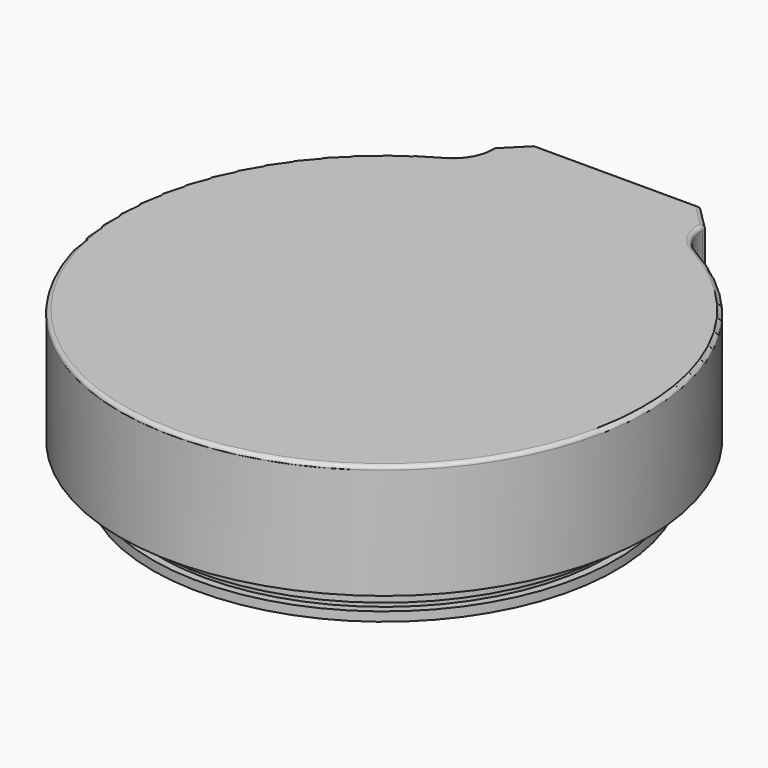
from build123d import *

# Parameters (mm, degrees)
F3_DEPTH      = 15
F4_R          = 30.35
F5_DEPTH      = 12
F8_DEPTH      = 5.2
F9_T1_DEPTH   = 15
F9_T6_DEPTH   = 27.1954073321
F9_S7_R       = 32.6
F9_T8_DEPTH   = 16
F9_S9_R       = 34.6
F9_T10_DEPTH  = 16
F9_T14_DEPTH  = 27.1954073321
F9_S15_R      = 32.6
F9_T16_DEPTH  = 16
F9_S17_R      = 34.6
F9_T18_DEPTH  = 16
F9_T23_DEPTH  = 27.1954073321
F9_S24_R      = 34.6
F9_T25_DEPTH  = 16
F9_T29_DEPTH  = 22.7968974984
F9_T37_DEPTH  = 27.1954073321
F9_S39_R      = 34.6
F9_T40_DEPTH  = 16
F9_T43_DEPTH  = 22.7968974984
F10_SIZE      = 3
F11_T1_DEPTH  = 24.2
F11_T3_DEPTH  = 6.7426406871
F11_T5_DEPTH  = 6.7426406871
F11_T7_DEPTH  = 1.6807325889
F11_T10_ANGLE = 303.1497240065
F11_T12_ANGLE = 61.5748620049
F11_T14_ANGLE = 61.5748620049


# Not quite as in the source:
# - a fillet or chamfer that OpenCascade refuses, or shapes differently, is made with other operations: its cross-section is extruded or revolved along the edge and cut away or added


with BuildPart() as f1:
    # F0 (on Front) → F1 (revolve)
    with BuildSketch(Plane.XZ):
        Polygon((-30.35, 1.2), (-30.35, 0), (-28.35, 0), (-28.35, 18.2), (0, 18.2), (0, 20.2), (-30.35, 20.2), (-32.6, 20.2), (-32.6, 8.2), (-30.35, 8.2), (-30.35, 5.2), (-29.35, 5.2), (-29.35, 4.2), (-30.35, 4.2), (-30.35, 2.2), (-29.35, 2.2), (-29.35, 1.2), align=None)
    revolve(axis=Axis((0, 0, 19.2), (0, 0, -1)))

    # F2 (on face) → F3 (join)
    with BuildSketch(Plane.XY.offset(20.2)):
        with BuildLine():
            Line((-13.85, 38.2565491622), (-13.85, 31.707057574))
            ThreePointArc((-13.85, 31.707057574), (0, -34.6), (13.85, 31.707057574))
            Line((13.85, 31.707057574), (13.85, 38.2565491622))
            Line((13.85, 38.2565491622), (-13.85, 38.2565491622))
        make_face()
        with BuildLine():
            ThreePointArc((11.85, 30.3700098782), (0, -32.6), (-11.85, 30.3700098782))
            Line((-11.85, 30.3700098782), (-11.85, 33.6700098782))
            Line((-11.85, 33.6700098782), (-9.35, 33.6700098782))
            Line((-9.35, 33.6700098782), (-9.35, 31.2303938496))
            ThreePointArc((-9.35, 31.2303938496), (0, 32.6), (9.35, 31.2303938496))
            Line((9.35, 31.2303938496), (9.35, 33.6700098782))
            Line((9.35, 33.6700098782), (11.85, 33.6700098782))
            Line((11.85, 33.6700098782), (11.85, 30.3700098782))
        make_face(mode=Mode.SUBTRACT)
    extrude(amount=-F3_DEPTH)

    # F4 (on face) → F5 (join)
    with BuildSketch(Plane(origin=(0, 0, 8.2), x_dir=(1, 0, 0), z_dir=(0, 0, -1))):
        with BuildLine():
            ThreePointArc((13.85, -31.707057574), (0, 34.6), (-13.85, -31.707057574))
            Line((-13.85, -31.707057574), (-13.85, -38.2565491622))
            Line((-13.85, -38.2565491622), (13.85, -38.2565491622))
            Line((13.85, -38.2565491622), (13.85, -31.707057574))
        make_face()
        Circle(F4_R, mode=Mode.SUBTRACT)
    extrude(amount=-F5_DEPTH)

    # F7 (on face) → F8 (join, through all)
    with BuildSketch(Plane(origin=(0, 0, 5.2), x_dir=(1, 0, 0), z_dir=(0, 0, -1))):
        with BuildLine():
            Line((-13.85, -29.5116502419), (-13.85, -38.2565491622))
            Line((-13.85, -38.2565491622), (13.85, -38.2565491622))
            Line((13.85, -38.2565491622), (13.85, -29.5116502419))
            ThreePointArc((13.85, -29.5116502419), (12.8571651353, -29.9575250093), (11.85, -30.3700098782))
            Line((11.85, -30.3700098782), (11.85, -33.6700098782))
            Line((11.85, -33.6700098782), (9.35, -33.6700098782))
            Line((9.35, -33.6700098782), (9.35, -31.2303938496))
            ThreePointArc((9.35, -31.2303938496), (0, -32.6), (-9.35, -31.2303938496))
            Line((-9.35, -31.2303938496), (-9.35, -33.6700098782))
            Line((-9.35, -33.6700098782), (-11.85, -33.6700098782))
            Line((-11.85, -33.6700098782), (-11.85, -30.3700098782))
            ThreePointArc((-11.85, -30.3700098782), (-12.8571651353, -29.9575250093), (-13.85, -29.5116502419))
        make_face()
    extrude(amount=F8_DEPTH)

    # F9: fillet of radius 5 on 4 edges, made by hand

    # F9_s2 → F9_t1 (join)
    with BuildSketch(Plane.XY.offset(5.2)):
        with BuildLine():
            ThreePointArc((-16.4699494949, 30.4286175111), (-14.5546389834, 32.2665444625), (-13.85, 34.8258165733))
            Line((-13.85, 34.8258165733), (-13.85, 31.707057574))
            ThreePointArc((-13.85, 31.707057574), (-15.1734451129, 31.0954428077), (-16.4699494949, 30.4286175111))
        make_face()
        with BuildLine():
            ThreePointArc((16.4699494949, 30.4286175111), (14.5546389834, 32.2665444625), (13.85, 34.8258165733))
            Line((13.85, 34.8258165733), (13.85, 31.707057574))
            ThreePointArc((13.85, 31.707057574), (15.1734451129, 31.0954428077), (16.4699494949, 30.4286175111))
        make_face()
    extrude(amount=F9_T1_DEPTH)


with BuildPart() as f9_tool4:
    # F9_s5 → F9_t6 (new body)
    with BuildSketch(Plane.XZ.offset(-44.207057574)):
        with BuildLine():
            ThreePointArc((13.85, 0.2), (15.3144660941, 3.7355339059), (18.85, 5.2))
            Line((18.85, 5.2), (13.85, 5.2))
            Line((13.85, 5.2), (13.85, 0.2))
        make_face()
    extrude(amount=F9_T6_DEPTH)

    # F9_s7 → F9_t8 (cut, symmetric)
    with BuildSketch(Plane.XY.offset(2.7)):
        Circle(F9_S7_R)
    extrude(amount=F9_T8_DEPTH, both=True, mode=Mode.SUBTRACT)

    # F9_s9 → F9_t10 (intersect, symmetric)
    with BuildSketch(Plane.XY.offset(2.7)):
        Circle(F9_S9_R)
    extrude(amount=F9_T10_DEPTH, both=True, mode=Mode.INTERSECT)


with BuildPart() as f1_1:
    add(f1.part)

    # F9_t3: union F9_tool4
    add(f9_tool4.part)


with BuildPart() as f9_tool12:
    # F9_s13 → F9_t14 (new body)
    with BuildSketch(Plane.XZ.offset(-17.0116502419)):
        with BuildLine():
            ThreePointArc((-18.85, 5.2), (-15.3144660941, 3.7355339059), (-13.85, 0.2))
            Line((-13.85, 0.2), (-13.85, 5.2))
            Line((-13.85, 5.2), (-18.85, 5.2))
        make_face()
    extrude(amount=-F9_T14_DEPTH)

    # F9_s15 → F9_t16 (cut, symmetric)
    with BuildSketch(Plane.XY.offset(2.7)):
        Circle(F9_S15_R)
    extrude(amount=F9_T16_DEPTH, both=True, mode=Mode.SUBTRACT)

    # F9_s17 → F9_t18 (intersect, symmetric)
    with BuildSketch(Plane.XY.offset(2.7)):
        Circle(F9_S17_R)
    extrude(amount=F9_T18_DEPTH, both=True, mode=Mode.INTERSECT)


with BuildPart() as f1_2:
    add(f1_1.part)

    # F9_t11: union F9_tool12
    add(f9_tool12.part)


with BuildPart() as f9_tool21:
    # F9_s22 → F9_t23 (new body)
    with BuildSketch(Plane.XZ.offset(-17.0116502419)):
        with BuildLine():
            ThreePointArc((-18.85, 5.2), (-15.3144660941, 3.7355339059), (-13.85, 0.2))
            Line((-13.85, 0.2), (-13.85, 5.2))
            Line((-13.85, 5.2), (-18.85, 5.2))
        make_face()
    extrude(amount=-F9_T23_DEPTH)

    # F9_s24 → F9_t25 (cut, symmetric)
    with BuildSketch(Plane.XY.offset(2.7)):
        Circle(F9_S24_R)
    extrude(amount=F9_T25_DEPTH, both=True, mode=Mode.SUBTRACT)

    split(bisect_by=Plane.XZ.offset(-38.2565491622), keep=Keep.TOP)


with BuildPart() as f9_tool27:
    # F9_s28 → F9_t29 (new body)
    with BuildSketch(Plane.XY.offset(-2.5968974984)):
        with BuildLine():
            ThreePointArc((-16.4699494949, 30.4286175111), (-14.5546389834, 32.2665444625), (-13.85, 34.8258165733))
            Line((-13.85, 34.8258165733), (-13.85, 31.707057574))
            ThreePointArc((-13.85, 31.707057574), (-15.1734451129, 31.0954428077), (-16.4699494949, 30.4286175111))
        make_face()
    extrude(amount=F9_T29_DEPTH)

    split(bisect_by=Plane.XY, keep=Keep.TOP)

    split(bisect_by=Plane.XY.offset(5.2), keep=Keep.BOTTOM)


with BuildPart() as f9_tool21_1:
    add(f9_tool21.part)

    # F9_t32: intersect F9_tool27
    add(f9_tool27.part, mode=Mode.INTERSECT)


with BuildPart() as f1_3:
    add(f1_2.part)

    # F9_t19: union F9_tool21
    add(f9_tool21_1.part)


with BuildPart() as f9_tool35:
    # F9_s36 → F9_t37 (new body)
    with BuildSketch(Plane.XZ.offset(-44.207057574)):
        with BuildLine():
            ThreePointArc((13.85, 0.2), (15.3144660941, 3.7355339059), (18.85, 5.2))
            Line((18.85, 5.2), (13.85, 5.2))
            Line((13.85, 5.2), (13.85, 0.2))
        make_face()
    extrude(amount=F9_T37_DEPTH)

    split(bisect_by=Plane.XZ.offset(-38.2565491622), keep=Keep.TOP)

    # F9_s39 → F9_t40 (cut, symmetric)
    with BuildSketch(Plane.XY.offset(2.7)):
        Circle(F9_S39_R)
    extrude(amount=F9_T40_DEPTH, both=True, mode=Mode.SUBTRACT)


with BuildPart() as f9_tool41:
    # F9_s42 → F9_t43 (new body)
    with BuildSketch(Plane.XY.offset(20.2)):
        with BuildLine():
            ThreePointArc((16.4699494949, 30.4286175111), (14.5546389834, 32.2665444625), (13.85, 34.8258165733))
            Line((13.85, 34.8258165733), (13.85, 31.707057574))
            ThreePointArc((13.85, 31.707057574), (15.1734451129, 31.0954428077), (16.4699494949, 30.4286175111))
        make_face()
    extrude(amount=-F9_T43_DEPTH)

    split(bisect_by=Plane.XY, keep=Keep.TOP)

    split(bisect_by=Plane.XY.offset(5.2), keep=Keep.BOTTOM)


with BuildPart() as f9_tool35_1:
    add(f9_tool35.part)

    # F9_t46: intersect F9_tool41
    add(f9_tool41.part, mode=Mode.INTERSECT)


with BuildPart() as f1_4:
    add(f1_3.part)

    # F9_t33: union F9_tool35
    add(f9_tool35_1.part)

    # F10
    f10_edges = [f1_4.edges().sort_by_distance(p)[0] for p in [
        (13.85, 38.256549, 12.7),
        (13.85, 38.256549, 2.6),
        (-13.85, 38.256549, 12.7),
        (-13.85, 38.256549, 2.6),
    ]]
    chamfer(f10_edges, length=F10_SIZE)

    # F11: fillet of radius 0.5 on 8 edges, made by hand

    # F11_s2 → F11_t1 (cut)
    with BuildSketch(Plane.YZ.offset(-12.1)):
        with BuildLine():
            ThreePointArc((38.2565491622, 19.7), (38.1101025528, 20.0535533906), (37.7565491622, 20.2))
            Line((37.7565491622, 20.2), (38.2565491622, 20.2))
            Line((38.2565491622, 20.2), (38.2565491622, 19.7))
        make_face()
    extrude(amount=F11_T1_DEPTH, mode=Mode.SUBTRACT)

    # F11_s4 → F11_t3 (cut)
    with BuildSketch(Plane(origin=(9.8193911046, 9.8193911046, 0), x_dir=(0, 0, 1), z_dir=(0.7071067812, 0.7071067812, 0))):
        with BuildLine():
            ThreePointArc((19.7, -34.7235739133), (20.0535533906, -34.5771273039), (20.2, -34.2235739133))
            Line((20.2, -34.2235739133), (20.2, -34.7235739133))
            Line((20.2, -34.7235739133), (19.7, -34.7235739133))
        make_face()
    extrude(amount=F11_T3_DEPTH, mode=Mode.SUBTRACT)

    # F11_s6 → F11_t5 (cut)
    with BuildSketch(Plane(origin=(-14.5871580576, 14.5871580576, 0), x_dir=(0, 0, 1), z_dir=(0.7071067812, -0.7071067812, 0))):
        with BuildLine():
            ThreePointArc((19.7, -34.7235739133), (20.0535533906, -34.5771273039), (20.2, -34.2235739133))
            Line((20.2, -34.2235739133), (20.2, -34.7235739133))
            Line((20.2, -34.7235739133), (19.7, -34.7235739133))
        make_face()
    extrude(amount=F11_T5_DEPTH, mode=Mode.SUBTRACT)

    # F11_s8 → F11_t7 (cut)
    with BuildSketch(Plane.XZ.offset(-36.5065491622)):
        with BuildLine():
            ThreePointArc((-13.85, 19.7), (-13.7035533906, 20.0535533906), (-13.35, 20.2))
            Line((-13.35, 20.2), (-13.85, 20.2))
            Line((-13.85, 20.2), (-13.85, 19.7))
        make_face()
        with BuildLine():
            ThreePointArc((13.85, 19.7), (13.7035533906, 20.0535533906), (13.35, 20.2))
            Line((13.35, 20.2), (13.85, 20.2))
            Line((13.85, 20.2), (13.85, 19.7))
        make_face()
    extrude(amount=F11_T7_DEPTH, mode=Mode.SUBTRACT)

    # F11_s9 → F11_t10 (revolve, cut)
    with BuildSketch(Plane(origin=(0, 0, 0), x_dir=(0, 0, 1), z_dir=(0.8794398125, 0.476010101, 0))):
        with BuildLine():
            ThreePointArc((20.2, -34.1), (20.0535533906, -34.4535533906), (19.7, -34.6))
            Line((19.7, -34.6), (20.2, -34.6))
            Line((20.2, -34.6), (20.2, -34.1))
        make_face()
    revolve(axis=Axis((0, 0, 20.2), (0, 0, 1)), revolution_arc=F11_T10_ANGLE, mode=Mode.SUBTRACT)

    # F11_s11 → F11_t12 (revolve, cut)
    with BuildSketch(Plane(origin=(-4e-10, -2e-10, 0), x_dir=(0, 0, 1), z_dir=(-0.8794398125, -0.476010101, 0))):
        with BuildLine():
            ThreePointArc((19.7, 34.6), (20.0535533906, 34.4535533906), (20.2, 34.1))
            Line((20.2, 34.1), (20.2, 34.6))
            Line((20.2, 34.6), (19.7, 34.6))
        make_face()
    revolve(axis=Axis((-18.8499999998, 34.8258165732, 20.2), (0, 0, 1)), revolution_arc=F11_T12_ANGLE, mode=Mode.SUBTRACT)

    # F11_s13 → F11_t14 (revolve, cut)
    with BuildSketch(Plane(origin=(4e-10, -2e-10, 0), x_dir=(0, 0, 1), z_dir=(0.8794398125, -0.476010101, 0))):
        with BuildLine():
            ThreePointArc((19.7, -34.6), (20.0535533906, -34.4535533906), (20.2, -34.1))
            Line((20.2, -34.1), (20.2, -34.6))
            Line((20.2, -34.6), (19.7, -34.6))
        make_face()
    revolve(axis=Axis((18.8499999998, 34.8258165732, 20.2), (0, 0, -1)), revolution_arc=F11_T14_ANGLE, mode=Mode.SUBTRACT)


solid = f1_4.part
